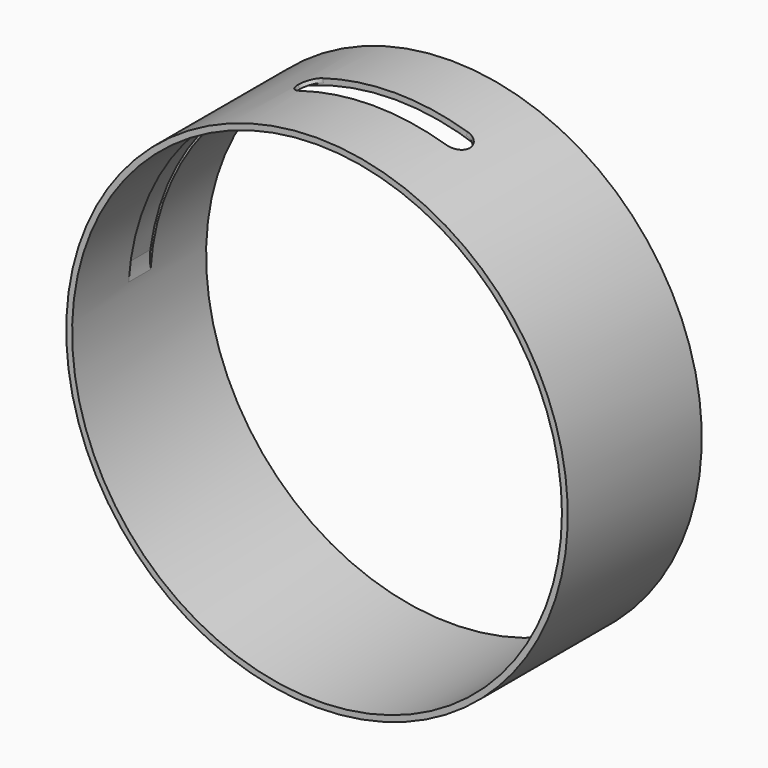
from build123d import *

# Parameters (mm, degrees)
F1_DEPTH = 107
F2_DEPTH = 17.5
F3_R     = 17.49999


# Not quite as in the source:
# - a fillet or chamfer is up to 0.001 mm smaller than in the source, because OpenCascade refuses the exact size


with BuildPart() as f1:
    # F0 (on Front) → F1 (new body, symmetric)
    with BuildSketch(Plane.XZ):
        with BuildLine():
            ThreePointArc((-109.6174559359, 301.1714849619), (-183.8312478505, -262.5382301946), (320.5, 0))
            ThreePointArc((320.5, 0), (262.5382301946, 183.8312478505), (109.6174559359, 301.1714849619))
            Line((109.6174559359, 301.1714849619), (107.9073522021, 296.4730135685))
            ThreePointArc((107.9073522021, 296.4730135685), (245.7106265432, 197.905362326), (312.6560960166, 42.2659444153))
            ThreePointArc((312.6560960166, 42.2659444153), (312.9876062183, 31.2398034738), (312.3457274768, 20.2273707381))
            ThreePointArc((312.3457274768, 20.2273707381), (312.836389108, 10.1189747444), (313, 0))
            ThreePointArc((313, 0), (-10.1189747444, -312.836389108), (-312.3457274768, 20.2273707381))
            ThreePointArc((-312.3457274768, 20.2273707381), (-312.9876062183, 31.2398034738), (-312.6560960166, 42.2659444153))
            ThreePointArc((-312.6560960166, 42.2659444153), (-245.7106265432, 197.905362326), (-107.9073522021, 296.4730135685))
            Line((-107.9073522021, 296.4730135685), (-109.6174559359, 301.1714849619))
        make_face()
        with BuildLine():
            Line((107.9073522021, 296.4730135685), (109.6174559359, 301.1714849619))
            ThreePointArc((109.6174559359, 301.1714849619), (55.6542409422, 315.6308848404), (0, 320.5))
            Line((0, 320.5), (0, 315.4999911785))
            ThreePointArc((0, 315.4999911785), (54.7859985221, 310.7068373879), (107.9073522021, 296.4730135685))
        make_face()
        with BuildLine():
            Line((-107.0523048609, 294.123790306), (-107.9073522021, 296.4730135685))
            ThreePointArc((-107.9073522021, 296.4730135685), (-245.7106265432, 197.905362326), (-312.6560960166, 42.2659444153))
            ThreePointArc((-312.6560960166, 42.2659444153), (-312.9876062183, 31.2398034738), (-312.3457274768, 20.2273707381))
            ThreePointArc((-312.3457274768, 20.2273707381), (-250.4565621924, 187.7245600735), (-107.0523048609, 294.123790306))
        make_face()
        with BuildLine():
            ThreePointArc((0, 320.5), (-55.6542409423, 315.6308848404), (-109.6174559359, 301.1714849619))
            Line((-109.6174559359, 301.1714849619), (-107.9073522021, 296.4730135685))
            ThreePointArc((-107.9073522021, 296.4730135685), (-54.7859985221, 310.7068373879), (0, 315.4999911785))
            Line((0, 315.4999911785), (0, 320.5))
        make_face()
        with BuildLine():
            ThreePointArc((312.6560960166, 42.2659444153), (245.7106265432, 197.905362326), (107.9073522021, 296.4730135685))
            Line((107.9073522021, 296.4730135685), (107.0523048609, 294.123790306))
            ThreePointArc((107.0523048609, 294.123790306), (250.4565621924, 187.7245600735), (312.3457274768, 20.2273707381))
            ThreePointArc((312.3457274768, 20.2273707381), (312.9876062183, 31.2398034738), (312.6560960166, 42.2659444153))
        make_face()
        with BuildLine():
            ThreePointArc((0, 315.4999911785), (-54.7859985221, 310.7068373879), (-107.9073522021, 296.4730135685))
            Line((-107.9073522021, 296.4730135685), (-107.0523048609, 294.123790306))
            ThreePointArc((-107.0523048609, 294.123790306), (-54.3518796098, 308.2448266928), (0, 313))
            Line((0, 313), (0, 315.4999911785))
        make_face()
        with BuildLine():
            Line((107.0523048609, 294.123790306), (107.9073522021, 296.4730135685))
            ThreePointArc((107.9073522021, 296.4730135685), (54.7859985221, 310.7068373879), (0, 315.4999911785))
            Line((0, 315.4999911785), (0, 313))
            ThreePointArc((0, 313), (54.3518796097, 308.2448266928), (107.0523048609, 294.123790306))
        make_face()
    extrude(amount=F1_DEPTH, both=True)

    # F0 (on Front) → F2 (cut, symmetric)
    with BuildSketch(Plane.XZ):
        with BuildLine():
            ThreePointArc((0, 320.5), (-55.6542409423, 315.6308848404), (-109.6174559359, 301.1714849619))
            Line((-109.6174559359, 301.1714849619), (-107.9073522021, 296.4730135685))
            ThreePointArc((-107.9073522021, 296.4730135685), (-54.7859985221, 310.7068373879), (0, 315.4999911785))
            Line((0, 315.4999911785), (0, 320.5))
        make_face()
        with BuildLine():
            Line((107.9073522021, 296.4730135685), (109.6174559359, 301.1714849619))
            ThreePointArc((109.6174559359, 301.1714849619), (55.6542409422, 315.6308848404), (0, 320.5))
            Line((0, 320.5), (0, 315.4999911785))
            ThreePointArc((0, 315.4999911785), (54.7859985221, 310.7068373879), (107.9073522021, 296.4730135685))
        make_face()
        with BuildLine():
            ThreePointArc((0, 315.4999911785), (-54.7859985221, 310.7068373879), (-107.9073522021, 296.4730135685))
            Line((-107.9073522021, 296.4730135685), (-107.0523048609, 294.123790306))
            ThreePointArc((-107.0523048609, 294.123790306), (-54.3518796098, 308.2448266928), (0, 313))
            Line((0, 313), (0, 315.4999911785))
        make_face()
        with BuildLine():
            Line((107.0523048609, 294.123790306), (107.9073522021, 296.4730135685))
            ThreePointArc((107.9073522021, 296.4730135685), (54.7859985221, 310.7068373879), (0, 315.4999911785))
            Line((0, 315.4999911785), (0, 313))
            ThreePointArc((0, 313), (54.3518796097, 308.2448266928), (107.0523048609, 294.123790306))
        make_face()
        with BuildLine():
            Line((-107.0523048609, 294.123790306), (-107.9073522021, 296.4730135685))
            ThreePointArc((-107.9073522021, 296.4730135685), (-245.7106265432, 197.905362326), (-312.6560960166, 42.2659444153))
            ThreePointArc((-312.6560960166, 42.2659444153), (-312.9876062183, 31.2398034738), (-312.3457274768, 20.2273707381))
            ThreePointArc((-312.3457274768, 20.2273707381), (-250.4565621924, 187.7245600735), (-107.0523048609, 294.123790306))
        make_face()
        with BuildLine():
            ThreePointArc((312.6560960166, 42.2659444153), (245.7106265432, 197.905362326), (107.9073522021, 296.4730135685))
            Line((107.9073522021, 296.4730135685), (107.0523048609, 294.123790306))
            ThreePointArc((107.0523048609, 294.123790306), (250.4565621924, 187.7245600735), (312.3457274768, 20.2273707381))
            ThreePointArc((312.3457274768, 20.2273707381), (312.9876062183, 31.2398034738), (312.6560960166, 42.2659444153))
        make_face()
    extrude(amount=F2_DEPTH, both=True, mode=Mode.SUBTRACT)

    # F3 (radius 17.5 in the source; OpenCascade refuses exactly that, so slightly less here)
    f3_edges = [f1.edges().sort_by_distance(p)[0] for p in [
        (-108.762404, 17.5, 298.822249),
        (108.762404, 17.5, 298.822249),
        (-108.762404, -17.5, 298.822249),
        (108.762404, -17.5, 298.822249),
    ]]
    fillet(f3_edges, radius=F3_R)


solid = f1.part
